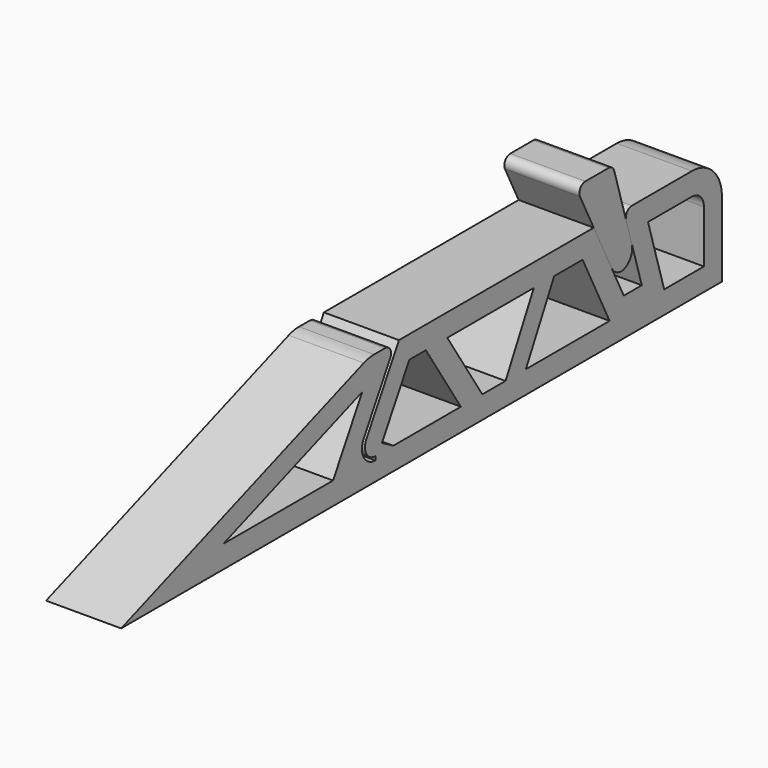
from build123d import *

# Parameters (mm, degrees)
F1_DEPTH     = 5
F2_R         = 5
F4_DEPTH     = 25
F6_DEPTH     = 10
F8_DEPTH     = 25
F9_R         = 1
F10_T1_DEPTH = 16.1803398875
F10_T3_DEPTH = 23.4403065089
F11_R        = 1


# Not quite as in the source:
# - a fillet or chamfer that OpenCascade refuses, or shapes differently, is made with other operations: its cross-section is extruded or revolved along the edge and cut away or added
# - ends of sketch curves that miss each other by under 0.0002 mm in the source are joined


with BuildPart() as f1:
    # F0 (on Right) → F1 (new body, symmetric)
    with BuildSketch(Plane.YZ):
        Polygon((-8.7878387082, 15), (-50, 0), (50, 0), (50, 15), align=None)
    extrude(amount=F1_DEPTH, both=True)

    # F2
    f2_edges = [f1.edges().sort_by_distance(p)[0] for p in [
        (0, 50, 15),
        (0, -8.787839, 15),
    ]]
    fillet(f2_edges, radius=F2_R)

    # F3 (on face) → F4 (cut)
    with BuildSketch(Plane.YZ.offset(5)):
        with BuildLine():
            Line((-3.7603476085, 15), (-4.3376978777, 15))
            Line((-4.3376978777, 15), (-9.6211402319, 5.8488094036))
            ThreePointArc((-9.6211402319, 5.8488094036), (-9.6211402319, 3.6128792242), (-7.6847678955, 2.4949141345))
            Line((-7.6847678955, 2.4949141345), (-7.6847678955, 2.9949141345))
            ThreePointArc((-7.6847678955, 2.9949141345), (-9.1871699303, 3.8612227218), (-9.190037249, 5.5954932374))
            Line((-9.190037249, 5.5954932374), (-3.7603476085, 15))
        make_face()
        Polygon((33.6602540378, 15), (28.6602540378, 15), (33.6602540378, 5), (36.6602540378, 5), align=None)
    extrude(amount=-F4_DEPTH, mode=Mode.SUBTRACT)

    # F7 (on face) → F8 (cut)
    with BuildSketch(Plane.YZ.offset(5)):
        Polygon((22.076485224, 12), (17.3679771944, 3), (31.3061520716, 3), (26.8061520716, 12), align=None)
        Polygon((4.2896619261, 12), (10.1192439169, 3), (13.9822219387, 3), (18.6907299683, 12), align=None)
        Polygon((-6.5919574173, 4.095507944), (-4.6944819983, 3), (6.5448904216, 3), (0.7153084307, 12), (-2.0282968009, 12), align=None)
        Polygon((-9.8730549791, 11.4124802622), (-32.9861545411, 3), (-14.7300027231, 3), align=None)
        with BuildLine():
            Line((45, 12), (37.6923459905, 12))
            Line((37.6923459905, 12), (40.3923459905, 3))
            Line((40.3923459905, 3), (47, 3))
            Line((47, 3), (47, 10))
            ThreePointArc((47, 10), (46.4142135624, 11.4142135624), (45, 12))
        make_face()
    extrude(amount=-F8_DEPTH, mode=Mode.SUBTRACT)

    # F9
    f9_edges = [f1.edges().sort_by_distance(p)[0] for p in [
        (0, -4.337698, 15),
        (0, 33.660254, 15),
    ]]
    fillet(f9_edges, radius=F9_R)


with BuildPart() as f6:
    # F5 (on face) → F6 (new body)
    with BuildSketch(Plane.YZ.offset(5)):
        Polygon((25.6602540378, 21), (32.1602540378, 8), (35.7602540378, 8), (31.8602540378, 21), align=None)
    extrude(amount=-F6_DEPTH)

    # F10: fillet of radius 2 on 2 edges, made by hand

    # F10_s2 → F10_t1 (cut)
    with BuildSketch(Plane.YZ.offset(-8.0901699437)):
        with BuildLine():
            ThreePointArc((31.6074676333, 9.105572809), (32.3448597911, 8.2986983833), (33.3963220153, 8))
            Line((33.3963220153, 8), (32.1602540378, 8))
            Line((32.1602540378, 8), (31.6074676333, 9.105572809))
        make_face()
    extrude(amount=F10_T1_DEPTH, mode=Mode.SUBTRACT)

    # F10_s4 → F10_t3 (cut)
    with BuildSketch(Plane.YZ.offset(-11.7201532545)):
        with BuildLine():
            ThreePointArc((33.0721927361, 8), (34.6767785926, 8.8061389407), (34.9878453065, 10.5746957711))
            Line((34.9878453065, 10.5746957711), (35.7602540378, 8))
            Line((35.7602540378, 8), (33.0721927361, 8))
        make_face()
    extrude(amount=F10_T3_DEPTH, mode=Mode.SUBTRACT)

    # F11
    f11_edges = [f6.edges().sort_by_distance(p)[0] for p in [
        (0, 25.660254, 21),
        (0, 31.860254, 21),
    ]]
    fillet(f11_edges, radius=F11_R)


solid = Compound([f1.part, f6.part])
